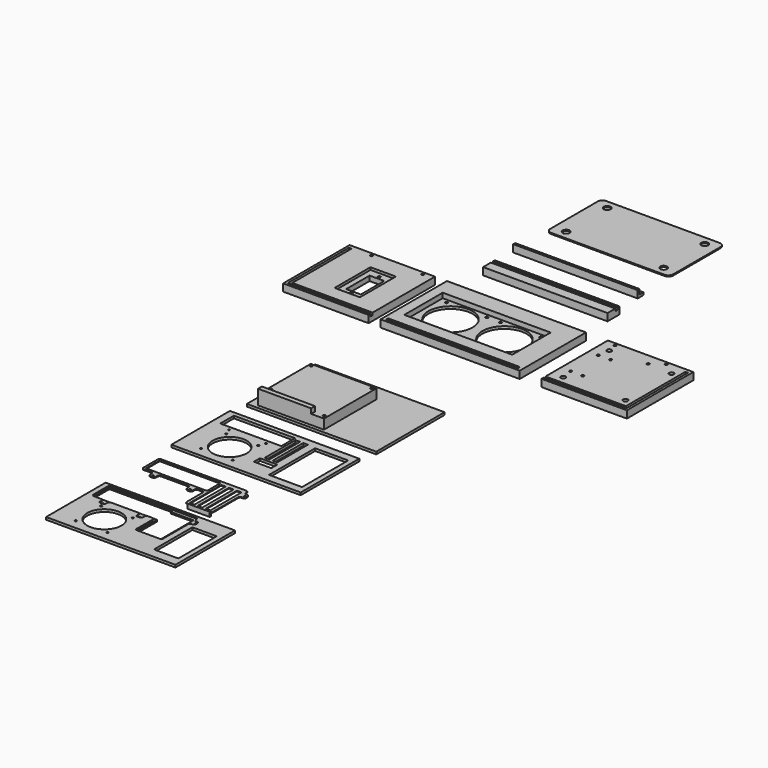
from build123d import *

# Parameters (mm, degrees)
F0_W      = 361.95
F0_H      = 215.9
F0_W_2    = 342.9
F0_H_2    = 6.731
F0_W_3    = 280.8
F0_H_3    = 125
F0_R      = 3.302
F0_R_2    = 57.5
F1_DEPTH  = 12.7
F2_DEPTH  = 6.35
F3_R      = 6
F3_R_2    = 3.302
F3_W      = 6.731
F3_H      = 3.556
F3_H_2    = 193.294
F4_DEPTH  = 12.7
F5_DEPTH  = 6.35
F6_R      = 3.302
F6_W      = 66.04
F6_H      = 116.84
F6_W_2    = 38.1
F6_H_2    = 76.2
F6_W_3    = 6.731
F6_H_3    = 193.294
F6_H_4    = 3.556
F7_DEPTH  = 12.7
F8_DEPTH  = 6.35
F9_DEPTH  = 6.35
F10_R     = 3.302
F10_W     = 138.0889187211
F10_H     = 12.6182494217
F11_DEPTH = 25.4
F12_DEPTH = 38.1
F13_R     = 3.302
F14_DEPTH = 6.4
F15_W     = 336.55
F15_H     = 190.385
F15_R     = 2.5
F15_R_2   = 44.5
F15_W_2   = 45.2000028
F15_H_2   = 20
F15_R_3   = 2.0970704069
F15_R_4   = 2.1817303996
F15_W_3   = 158.75
F15_H_3   = 44.45
F15_W_4   = 12.0000014
F15_H_4   = 99.38
F15_W_5   = 86
F15_H_5   = 150
F16_DEPTH = 6.3754
F17_W     = 323.85
F17_H     = 25.2222
F17_H_2   = 6.5278
F17_H_3   = 6.35
F18_DEPTH = 12.7
F19_DEPTH = 6.35
F20_R     = 9
F21_DEPTH = 3
F22_DEPTH = 6.35
F23_R     = 2
F23_W     = 158.75
F23_H     = 44.45
F24_DEPTH = 2
F25_DEPTH = 10
F26_W     = 336.55
F26_H     = 193.6500064
F26_R     = 2.5
F26_R_2   = 44.5
F26_W_2   = 63.5
F26_H_2   = 125
F26_R_3   = 2
F27_DEPTH = 6.4
F28_START = 4
F28_DEPTH = 2.4
F29_W     = 323.85
F29_H     = 6.35
F30_DEPTH = 19.05
F29_H_2   = 12.7
F31_DEPTH = 6.35


# Not quite as in the source:
# - a feature names something its author has since deleted; it is built from what else it names


with BuildPart() as f1:
    # F0 (on Top) → F1 (new body)
    with BuildSketch(Plane.XY):
        with Locations((-60.325, 0)):
            Rectangle(F0_W, F0_H)
        with Locations((-60.325, -98.2345)):
            Rectangle(F0_W_2, F0_H_2, mode=Mode.SUBTRACT)
        with Locations((-75.5, 0)):
            Rectangle(F0_W_3, F0_H_3, mode=Mode.SUBTRACT)
        with Locations((-60.325, -98.2345)):
            Rectangle(F0_W_2, F0_H_2)
        with Locations((-75.5, 0)):
            Rectangle(F0_W_3, F0_H_3)
        with Locations((-198.2, -52.5)):
            Circle(F0_R, mode=Mode.SUBTRACT)
        with Locations((-93.2, -52.5)):
            Circle(F0_R, mode=Mode.SUBTRACT)
        with Locations((-57.8, -52.5)):
            Circle(F0_R, mode=Mode.SUBTRACT)
        with Locations((47.2, -52.5)):
            Circle(F0_R, mode=Mode.SUBTRACT)
        with Locations((-198.2, 52.5)):
            Circle(F0_R, mode=Mode.SUBTRACT)
        with Locations((-145.7, 0)):
            Circle(F0_R_2, mode=Mode.SUBTRACT)
        with Locations((-93.2, 52.5)):
            Circle(F0_R, mode=Mode.SUBTRACT)
        with Locations((-5.3, 0)):
            Circle(F0_R_2, mode=Mode.SUBTRACT)
        with Locations((-57.8, 52.5)):
            Circle(F0_R, mode=Mode.SUBTRACT)
        with Locations((47.2, 52.5)):
            Circle(F0_R, mode=Mode.SUBTRACT)
    extrude(amount=-F1_DEPTH)

    # F0 (on Top) → F2 (join)
    with BuildSketch(Plane.XY):
        with Locations((-60.325, 0)):
            Rectangle(F0_W, F0_H)
        with Locations((-60.325, -98.2345)):
            Rectangle(F0_W_2, F0_H_2, mode=Mode.SUBTRACT)
        with Locations((-75.5, 0)):
            Rectangle(F0_W_3, F0_H_3, mode=Mode.SUBTRACT)
        with Locations((-75.5, 0)):
            Rectangle(F0_W_3, F0_H_3)
        with Locations((-198.2, -52.5)):
            Circle(F0_R, mode=Mode.SUBTRACT)
        with Locations((-93.2, -52.5)):
            Circle(F0_R, mode=Mode.SUBTRACT)
        with Locations((-57.8, -52.5)):
            Circle(F0_R, mode=Mode.SUBTRACT)
        with Locations((47.2, -52.5)):
            Circle(F0_R, mode=Mode.SUBTRACT)
        with Locations((-198.2, 52.5)):
            Circle(F0_R, mode=Mode.SUBTRACT)
        with Locations((-145.7, 0)):
            Circle(F0_R_2, mode=Mode.SUBTRACT)
        with Locations((-93.2, 52.5)):
            Circle(F0_R, mode=Mode.SUBTRACT)
        with Locations((-5.3, 0)):
            Circle(F0_R_2, mode=Mode.SUBTRACT)
        with Locations((-57.8, 52.5)):
            Circle(F0_R, mode=Mode.SUBTRACT)
        with Locations((47.2, 52.5)):
            Circle(F0_R, mode=Mode.SUBTRACT)
    extrude(amount=F2_DEPTH)

    # F0 (on Top) → F22 (cut, symmetric)
    with BuildSketch(Plane.XY):
        with Locations((-75.5, 0)):
            Rectangle(F0_W_3, F0_H_3)
        with Locations((-198.2, -52.5)):
            Circle(F0_R, mode=Mode.SUBTRACT)
        with Locations((-93.2, -52.5)):
            Circle(F0_R, mode=Mode.SUBTRACT)
        with Locations((-57.8, -52.5)):
            Circle(F0_R, mode=Mode.SUBTRACT)
        with Locations((47.2, -52.5)):
            Circle(F0_R, mode=Mode.SUBTRACT)
        with Locations((-198.2, 52.5)):
            Circle(F0_R, mode=Mode.SUBTRACT)
        with Locations((-145.7, 0)):
            Circle(F0_R_2, mode=Mode.SUBTRACT)
        with Locations((-93.2, 52.5)):
            Circle(F0_R, mode=Mode.SUBTRACT)
        with Locations((-5.3, 0)):
            Circle(F0_R_2, mode=Mode.SUBTRACT)
        with Locations((-57.8, 52.5)):
            Circle(F0_R, mode=Mode.SUBTRACT)
        with Locations((47.2, 52.5)):
            Circle(F0_R, mode=Mode.SUBTRACT)
    extrude(amount=F22_DEPTH, both=True, mode=Mode.SUBTRACT)


with BuildPart() as f4:
    # F3 (on Top) → F4 (new body)
    with BuildSketch(Plane.XY):
        Polygon((177.3511743546, -101.6), (177.3511743546, -107.95), (399.6011743546, -107.95), (399.6011743546, 107.95), (177.3511743546, 107.95), (177.3511743546, -94.869), (386.5201743546, -94.869), (386.5201743546, 98.425), (393.2511743546, 98.425), (393.2511743546, -94.869), (393.2511743546, -98.425), (393.2511743546, -101.6), align=None)
        with Locations((207.3511743546, -74.95)):
            Circle(F3_R, mode=Mode.SUBTRACT)
        with BuildLine():
            Line((231.2492377546, -45.0850025), (206.0531743546, -45.0850025))
            ThreePointArc((206.0531743546, -45.0850025), (200.4163077631, -47.4198690915), (202.7511743546, -41.7830025))
            Line((202.7511743546, -41.7830025), (202.7511743546, 41.7829975))
            ThreePointArc((202.7511743546, 41.7829975), (200.4163077631, 47.4198640915), (206.0531743546, 45.0849975))
            Line((206.0531743546, 45.0849975), (231.2492377546, 45.0849975))
            ThreePointArc((231.2492377546, 45.0849975), (234.5512377546, 48.3869975), (237.8532377546, 45.0849975))
            ThreePointArc((237.8532377546, 45.0849975), (236.886104346, 42.7501309085), (234.5512377546, 41.7829975))
            Line((234.5512377546, 41.7829975), (234.5512377546, -41.7830025))
            ThreePointArc((234.5512377546, -41.7830025), (236.886104346, -42.7501359085), (237.8532377546, -45.0850025))
            ThreePointArc((237.8532377546, -45.0850025), (234.5512377546, -48.3870025), (231.2492377546, -45.0850025))
        make_face(mode=Mode.SUBTRACT)
        with Locations((369.6011743546, -74.95)):
            Circle(F3_R, mode=Mode.SUBTRACT)
        with Locations((207.3511743546, 74.95)):
            Circle(F3_R, mode=Mode.SUBTRACT)
        with Locations((202.7511743546, 99.95)):
            Circle(F3_R_2, mode=Mode.SUBTRACT)
        with Locations((306.0201743546, 78.45)):
            Circle(F3_R_2, mode=Mode.SUBTRACT)
        with Locations((335.8979743546, 99.95)):
            Circle(F3_R_2, mode=Mode.SUBTRACT)
        with Locations((369.6011743546, 74.95)):
            Circle(F3_R, mode=Mode.SUBTRACT)
        Polygon((177.3511743546, -94.869), (177.3511743546, -101.6), (393.2511743546, -101.6), (393.2511743546, -98.425), (386.5201743546, -98.425), (386.5201743546, -94.869), align=None)
        with Locations((389.8856743546, -96.647)):
            Rectangle(F3_W, F3_H)
        with Locations((389.8856743546, 1.778)):
            Rectangle(F3_W, F3_H_2)
        with Locations((207.3511743546, 74.95)):
            Circle(F3_R)
        with Locations((207.3511743546, 74.95)):
            Circle(F3_R_2, mode=Mode.SUBTRACT)
        with Locations((207.3511743546, -74.95)):
            Circle(F3_R)
        with Locations((207.3511743546, -74.95)):
            Circle(F3_R_2, mode=Mode.SUBTRACT)
        with Locations((369.6011743546, -74.95)):
            Circle(F3_R)
        with Locations((369.6011743546, -74.95)):
            Circle(F3_R_2, mode=Mode.SUBTRACT)
        with Locations((369.6011743546, 74.95)):
            Circle(F3_R)
        with Locations((369.6011743546, 74.95)):
            Circle(F3_R_2, mode=Mode.SUBTRACT)
        with BuildLine():
            ThreePointArc((202.7511743546, -41.7830025), (205.086040946, -42.7501359085), (206.0531743546, -45.0850025))
            Line((206.0531743546, -45.0850025), (231.2492377546, -45.0850025))
            ThreePointArc((231.2492377546, -45.0850025), (232.2163711631, -42.7501359085), (234.5512377546, -41.7830025))
            Line((234.5512377546, -41.7830025), (234.5512377546, 41.7829975))
            ThreePointArc((234.5512377546, 41.7829975), (232.2163711631, 42.7501309085), (231.2492377546, 45.0849975))
            Line((231.2492377546, 45.0849975), (206.0531743546, 45.0849975))
            ThreePointArc((206.0531743546, 45.0849975), (205.086040946, 42.7501309085), (202.7511743546, 41.7829975))
            Line((202.7511743546, 41.7829975), (202.7511743546, -41.7830025))
        make_face()
    extrude(amount=-F4_DEPTH)

    # F3 (on Top) → F5 (join)
    with BuildSketch(Plane.XY):
        Polygon((177.3511743546, -101.6), (177.3511743546, -107.95), (399.6011743546, -107.95), (399.6011743546, 107.95), (177.3511743546, 107.95), (177.3511743546, -94.869), (386.5201743546, -94.869), (386.5201743546, 98.425), (393.2511743546, 98.425), (393.2511743546, -94.869), (393.2511743546, -98.425), (393.2511743546, -101.6), align=None)
        with Locations((207.3511743546, -74.95)):
            Circle(F3_R, mode=Mode.SUBTRACT)
        with BuildLine():
            Line((231.2492377546, -45.0850025), (206.0531743546, -45.0850025))
            ThreePointArc((206.0531743546, -45.0850025), (200.4163077631, -47.4198690915), (202.7511743546, -41.7830025))
            Line((202.7511743546, -41.7830025), (202.7511743546, 41.7829975))
            ThreePointArc((202.7511743546, 41.7829975), (200.4163077631, 47.4198640915), (206.0531743546, 45.0849975))
            Line((206.0531743546, 45.0849975), (231.2492377546, 45.0849975))
            ThreePointArc((231.2492377546, 45.0849975), (234.5512377546, 48.3869975), (237.8532377546, 45.0849975))
            ThreePointArc((237.8532377546, 45.0849975), (236.886104346, 42.7501309085), (234.5512377546, 41.7829975))
            Line((234.5512377546, 41.7829975), (234.5512377546, -41.7830025))
            ThreePointArc((234.5512377546, -41.7830025), (236.886104346, -42.7501359085), (237.8532377546, -45.0850025))
            ThreePointArc((237.8532377546, -45.0850025), (234.5512377546, -48.3870025), (231.2492377546, -45.0850025))
        make_face(mode=Mode.SUBTRACT)
        with Locations((369.6011743546, -74.95)):
            Circle(F3_R, mode=Mode.SUBTRACT)
        with Locations((207.3511743546, 74.95)):
            Circle(F3_R, mode=Mode.SUBTRACT)
        with Locations((202.7511743546, 99.95)):
            Circle(F3_R_2, mode=Mode.SUBTRACT)
        with Locations((306.0201743546, 78.45)):
            Circle(F3_R_2, mode=Mode.SUBTRACT)
        with Locations((335.8979743546, 99.95)):
            Circle(F3_R_2, mode=Mode.SUBTRACT)
        with Locations((369.6011743546, 74.95)):
            Circle(F3_R, mode=Mode.SUBTRACT)
        with BuildLine():
            ThreePointArc((202.7511743546, -41.7830025), (205.086040946, -42.7501359085), (206.0531743546, -45.0850025))
            Line((206.0531743546, -45.0850025), (231.2492377546, -45.0850025))
            ThreePointArc((231.2492377546, -45.0850025), (232.2163711631, -42.7501359085), (234.5512377546, -41.7830025))
            Line((234.5512377546, -41.7830025), (234.5512377546, 41.7829975))
            ThreePointArc((234.5512377546, 41.7829975), (232.2163711631, 42.7501309085), (231.2492377546, 45.0849975))
            Line((231.2492377546, 45.0849975), (206.0531743546, 45.0849975))
            ThreePointArc((206.0531743546, 45.0849975), (205.086040946, 42.7501309085), (202.7511743546, 41.7829975))
            Line((202.7511743546, 41.7829975), (202.7511743546, -41.7830025))
        make_face()
    extrude(amount=F5_DEPTH)


with BuildPart() as f7:
    # F6 (on Top) → F7 (new body)
    with BuildSketch(Plane.XY):
        Polygon((-272.3593753815, -94.869), (-272.3593753815, 107.95), (-494.6093753815, 107.95), (-494.6093753815, -107.95), (-272.3593753815, -107.95), (-272.3593753815, -101.6), (-488.2593753815, -101.6), (-488.2593753815, -98.425), (-488.2593753815, -94.869), (-488.2593753815, 98.425), (-481.5283753815, 98.425), (-481.5283753815, -94.869), align=None)
        with Locations((-430.9061753815, 99.95)):
            Circle(F6_R, mode=Mode.SUBTRACT)
        with Locations((-367.6093753815, 0)):
            Rectangle(F6_W, F6_H, mode=Mode.SUBTRACT)
        with Locations((-297.7593753815, 99.95)):
            Circle(F6_R, mode=Mode.SUBTRACT)
        with Locations((-367.6093753815, 0)):
            Rectangle(F6_W, F6_H)
        with Locations((-367.6093753815, -45.6)):
            Circle(F6_R, mode=Mode.SUBTRACT)
        with Locations((-367.6093753815, 0)):
            Rectangle(F6_W_2, F6_H_2, mode=Mode.SUBTRACT)
        with Locations((-367.6093753815, 45.6)):
            Circle(F6_R, mode=Mode.SUBTRACT)
        Polygon((-272.3593753815, -101.6), (-272.3593753815, -94.869), (-481.5283753815, -94.869), (-481.5283753815, -98.425), (-488.2593753815, -98.425), (-488.2593753815, -101.6), align=None)
        with Locations((-484.8938753815, 1.778)):
            Rectangle(F6_W_3, F6_H_3)
        with Locations((-484.8938753815, -96.647)):
            Rectangle(F6_W_3, F6_H_4)
    extrude(amount=-F7_DEPTH)

    # F6 (on Top) → F8 (join)
    with BuildSketch(Plane.XY):
        Polygon((-272.3593753815, -94.869), (-272.3593753815, 107.95), (-494.6093753815, 107.95), (-494.6093753815, -107.95), (-272.3593753815, -107.95), (-272.3593753815, -101.6), (-488.2593753815, -101.6), (-488.2593753815, -98.425), (-488.2593753815, -94.869), (-488.2593753815, 98.425), (-481.5283753815, 98.425), (-481.5283753815, -94.869), align=None)
        with Locations((-430.9061753815, 99.95)):
            Circle(F6_R, mode=Mode.SUBTRACT)
        with Locations((-367.6093753815, 0)):
            Rectangle(F6_W, F6_H, mode=Mode.SUBTRACT)
        with Locations((-297.7593753815, 99.95)):
            Circle(F6_R, mode=Mode.SUBTRACT)
        with Locations((-367.6093753815, 0)):
            Rectangle(F6_W, F6_H)
        with Locations((-367.6093753815, -45.6)):
            Circle(F6_R, mode=Mode.SUBTRACT)
        with Locations((-367.6093753815, 0)):
            Rectangle(F6_W_2, F6_H_2, mode=Mode.SUBTRACT)
        with Locations((-367.6093753815, 45.6)):
            Circle(F6_R, mode=Mode.SUBTRACT)
    extrude(amount=F8_DEPTH)

    # F6 (on Top) → F9 (cut)
    with BuildSketch(Plane.XY):
        with Locations((-367.6093753815, 0)):
            Rectangle(F6_W, F6_H)
        with Locations((-367.6093753815, -45.6)):
            Circle(F6_R, mode=Mode.SUBTRACT)
        with Locations((-367.6093753815, 0)):
            Rectangle(F6_W_2, F6_H_2, mode=Mode.SUBTRACT)
        with Locations((-367.6093753815, 45.6)):
            Circle(F6_R, mode=Mode.SUBTRACT)
    extrude(amount=F9_DEPTH, mode=Mode.SUBTRACT)


with BuildPart() as f11:
    # F10 (on Top) → F11 (new body)
    with BuildSketch(Plane.XY):
        Polygon((-35.35, -549.4468963333), (-35.35, -377.9968963333), (-206.8, -377.9968963333), (-206.8, -536.8286469116), (-68.7110812789, -536.8286469116), (-68.7110812789, -549.4468963333), align=None)
        with Locations((-200.45, -516.4268963333)):
            Circle(F10_R, mode=Mode.SUBTRACT)
        with Locations((-42.97, -539.2868963333)):
            Circle(F10_R, mode=Mode.SUBTRACT)
        with Locations((-200.45, -384.3468963333)):
            Circle(F10_R, mode=Mode.SUBTRACT)
        with Locations((-42.97, -384.3468963333)):
            Circle(F10_R, mode=Mode.SUBTRACT)
        with Locations((-137.7555406395, -543.1377716225)):
            Rectangle(F10_W, F10_H)
    extrude(amount=F11_DEPTH)

    # F10 (on Top) → F12 (join)
    with BuildSketch(Plane.XY):
        with Locations((-137.7555406395, -543.1377716225)):
            Rectangle(F10_W, F10_H)
    extrude(amount=F12_DEPTH)


with BuildPart() as f14:
    # F13 (on Top) → F14 (new body)
    with BuildSketch(Plane.XY):
        Polygon((107.95, -558.4746963333), (107.95, -336.2246963333), (-228.6, -336.2246963333), (-228.6, -551.9468963333), (-228.6, -558.4746963333), align=None)
        with Locations((-200.45, -516.4268963333)):
            Circle(F13_R, mode=Mode.SUBTRACT)
        with Locations((-42.97, -539.2868963333)):
            Circle(F13_R, mode=Mode.SUBTRACT)
        with Locations((-200.45, -384.3468963333)):
            Circle(F13_R, mode=Mode.SUBTRACT)
        with Locations((-42.97, -384.3468963333)):
            Circle(F13_R, mode=Mode.SUBTRACT)
    extrude(amount=-F14_DEPTH)


with BuildPart() as f16:
    # F15 (on Top) → F16 (new body)
    with BuildSketch(Plane.XY):
        with Locations((-60.325, -708.9570045471)):
            Rectangle(F15_W, F15_H)
        with Locations((-171.0694, -779.3595045471)):
            Circle(F15_R, mode=Mode.SUBTRACT)
        with Locations((-88.5694, -779.3595045471)):
            Circle(F15_R, mode=Mode.SUBTRACT)
        with Locations((-129.8194, -738.1095045471)):
            Circle(F15_R_2, mode=Mode.SUBTRACT)
        with Locations((-28.20002274, -747.9644930071)):
            Rectangle(F15_W_2, F15_H_2, mode=Mode.SUBTRACT)
        with Locations((-171.0694, -696.8595045471)):
            Circle(F15_R, mode=Mode.SUBTRACT)
        with Locations((-177.92501754, -679.9145094071)):
            Circle(F15_R_3, mode=Mode.SUBTRACT)
        with Locations((-88.5694, -696.8595045471)):
            Circle(F15_R, mode=Mode.SUBTRACT)
        with Locations((-81.72500674, -679.9145094071)):
            Circle(F15_R_4, mode=Mode.SUBTRACT)
        with Locations((-129.82501214, -647.1895050071)):
            Rectangle(F15_W_3, F15_H_3, mode=Mode.SUBTRACT)
        with Locations((-38.45002344, -680.6544930071)):
            Rectangle(F15_W_4, F15_H_4, mode=Mode.SUBTRACT)
        with Locations((-17.95002204, -680.6544930071)):
            Rectangle(F15_W_4, F15_H_4, mode=Mode.SUBTRACT)
        with Locations((52.25, -708.9570045471)):
            Rectangle(F15_W_5, F15_H_5, mode=Mode.SUBTRACT)
    extrude(amount=F16_DEPTH)


with BuildPart() as f18:
    # F17 (on Top) → F18 (new body)
    with BuildSketch(Plane.XY):
        with Locations((-60.325, 214.3075841795)):
            Rectangle(F17_W, F17_H)
        with Locations((-60.325, 230.1825841795)):
            Rectangle(F17_W, F17_H_2)
        with Locations((-60.325, 236.6214841795)):
            Rectangle(F17_W, F17_H_3)
    extrude(amount=-F18_DEPTH)

    # F17 (on Top) → F19 (join)
    with BuildSketch(Plane.XY):
        with Locations((-60.325, 236.6214841795)):
            Rectangle(F17_W, F17_H_3)
        with Locations((-60.325, 214.3075841795)):
            Rectangle(F17_W, F17_H)
    extrude(amount=F19_DEPTH)


with BuildPart() as f21:
    # F20 (on Top) → F21 (new body)
    with BuildSketch(Plane.XY):
        with BuildLine():
            ThreePointArc((-224.79, 423.5097664064), (-221.0702561211, 414.5295102853), (-212.09, 410.8097664064))
            Line((-212.09, 410.8097664064), (82.4, 410.8097664064))
            ThreePointArc((82.4, 410.8097664064), (91.3802561211, 414.5295102853), (95.1, 423.5097664064))
            Line((95.1, 423.5097664064), (95.1, 577.3067664064))
            ThreePointArc((95.1, 577.3067664064), (91.3802561211, 586.2870225275), (82.4, 590.0067664064))
            Line((82.4, 590.0067664064), (-212.09, 590.0067664064))
            ThreePointArc((-212.09, 590.0067664064), (-221.0702561211, 586.2870225275), (-224.79, 577.3067664064))
            Line((-224.79, 577.3067664064), (-224.79, 423.5097664064))
        make_face()
        with Locations((-191.77, 433.6697664064)):
            Circle(F20_R, mode=Mode.SUBTRACT)
        with Locations((62.08, 433.6697664064)):
            Circle(F20_R, mode=Mode.SUBTRACT)
        with Locations((-191.77, 567.1467664064)):
            Circle(F20_R, mode=Mode.SUBTRACT)
        with Locations((62.08, 567.1467664064)):
            Circle(F20_R, mode=Mode.SUBTRACT)
    extrude(amount=F21_DEPTH)


with BuildPart() as f24:
    # F23 (on Top) → F24 (new body)
    with BuildSketch(Plane.XY):
        with BuildLine():
            Line((-3.45002134, -872.449751843), (8.54998006, -872.449751843))
            Line((8.54998006, -872.449751843), (8.54998006, -974.0499811521))
            Line((8.54998006, -974.0499811521), (11.08998006, -974.0499811521))
            Line((11.08998006, -974.0499811521), (11.08998006, -979.449751843))
            Line((11.08998006, -979.449751843), (11.46998006, -979.449751843))
            ThreePointArc((11.46998006, -979.449751843), (15.0620825084, -977.9618542914), (16.54998006, -974.369751843))
            Line((16.54998006, -974.369751843), (16.54998006, -893.4699931521))
            ThreePointArc((16.54998006, -893.4699931521), (18.0378776116, -889.8778907037), (21.62998006, -888.3899931521))
            Line((21.62998006, -888.3899931521), (24.16998006, -888.3899931521))
            ThreePointArc((24.16998006, -888.3899931521), (27.7620825084, -886.9020956005), (29.24998006, -883.3099931521))
            Line((29.24998006, -883.3099931521), (29.24998006, -878.2299931521))
            ThreePointArc((29.24998006, -878.2299931521), (27.7620825084, -874.6378907037), (24.16998006, -873.1499931521))
            Line((24.16998006, -873.1499931521), (21.62998006, -873.1499931521))
            ThreePointArc((21.62998006, -873.1499931521), (18.0378776116, -871.6620956005), (16.54998006, -868.0699931521))
            Line((16.54998006, -868.0699931521), (16.54998006, -865.5299931521))
            ThreePointArc((16.54998006, -865.5299931521), (15.0620825084, -861.9378907037), (11.46998006, -860.4499931521))
            Line((11.46998006, -860.4499931521), (-210.12001214, -860.4499931521))
            ThreePointArc((-210.12001214, -860.4499931521), (-213.7121145884, -861.9378907037), (-215.20001214, -865.5299931521))
            Line((-215.20001214, -865.5299931521), (-215.20001214, -911.8199931521))
            ThreePointArc((-215.20001214, -911.8199931521), (-213.7121145884, -915.4120956005), (-210.12001214, -916.8999931521))
            Line((-210.12001214, -916.8999931521), (-190.62501754, -916.8999931521))
            ThreePointArc((-190.62501754, -916.8999931521), (-187.0329150916, -918.3878907037), (-185.54501754, -921.9799931521))
            Line((-185.54501754, -921.9799931521), (-185.54501754, -927.0599931521))
            ThreePointArc((-185.54501754, -927.0599931521), (-184.0571199884, -930.6520956005), (-180.46501754, -932.1399931521))
            Line((-180.46501754, -932.1399931521), (-175.38501754, -932.1399931521))
            ThreePointArc((-175.38501754, -932.1399931521), (-171.7929150916, -930.6520956005), (-170.30501754, -927.0599931521))
            Line((-170.30501754, -927.0599931521), (-170.30501754, -921.9799931521))
            ThreePointArc((-170.30501754, -921.9799931521), (-168.8171199884, -918.3878907037), (-165.22501754, -916.8999931521))
            Line((-165.22501754, -916.8999931521), (-94.42500674, -916.8999931521))
            ThreePointArc((-94.42500674, -916.8999931521), (-90.8329042916, -918.3878907037), (-89.34500674, -921.9799931521))
            Line((-89.34500674, -921.9799931521), (-89.34500674, -927.0599931521))
            ThreePointArc((-89.34500674, -927.0599931521), (-87.8571091884, -930.6520956005), (-84.26500674, -932.1399931521))
            Line((-84.26500674, -932.1399931521), (-79.18500674, -932.1399931521))
            ThreePointArc((-79.18500674, -932.1399931521), (-75.5929042916, -930.6520956005), (-74.10500674, -927.0599931521))
            Line((-74.10500674, -927.0599931521), (-74.10500674, -921.9799931521))
            ThreePointArc((-74.10500674, -921.9799931521), (-72.6171091884, -918.3878907037), (-69.02500674, -916.8999931521))
            Line((-69.02500674, -916.8999931521), (-57.53002414, -916.8999931521))
            ThreePointArc((-57.53002414, -916.8999931521), (-53.9379216916, -918.3878907037), (-52.45002414, -921.9799931521))
            Line((-52.45002414, -921.9799931521), (-52.45002414, -974.369751843))
            ThreePointArc((-52.45002414, -974.369751843), (-50.9621265884, -977.9618542914), (-47.37002414, -979.449751843))
            Line((-47.37002414, -979.449751843), (-46.99002414, -979.449751843))
            Line((-46.99002414, -979.449751843), (-46.99002414, -974.0499811521))
            Line((-46.99002414, -974.0499811521), (-44.45002414, -974.0499811521))
            Line((-44.45002414, -974.0499811521), (-44.45002414, -872.4499811521))
            Line((-44.45002414, -872.4499811521), (-32.45002274, -872.4499811521))
            Line((-32.45002274, -872.4499811521), (-32.45002274, -974.0499811521))
            Line((-32.45002274, -974.0499811521), (-23.95002274, -974.0499811521))
            Line((-23.95002274, -974.0499811521), (-23.95002274, -872.4499811521))
            Line((-23.95002274, -872.4499811521), (-11.95002134, -872.4499811521))
            Line((-11.95002134, -872.4499811521), (-11.95002134, -974.0499811521))
            Line((-11.95002134, -974.0499811521), (-3.45002134, -974.0499811521))
            Line((-3.45002134, -974.0499811521), (-3.45002134, -872.449751843))
        make_face()
        with Locations((-177.92501754, -927.4099931521)):
            Circle(F23_R, mode=Mode.SUBTRACT)
        with Locations((-81.72500674, -927.4099931521)):
            Circle(F23_R, mode=Mode.SUBTRACT)
        with Locations((-129.82501214, -888.6749931521)):
            Rectangle(F23_W, F23_H, mode=Mode.SUBTRACT)
        with Locations((24.51999206, -880.7699931521)):
            Circle(F23_R, mode=Mode.SUBTRACT)
        Polygon((11.08998006, -974.0499811521), (8.54998006, -974.0499811521), (-3.45002134, -974.0499811521), (-11.95002134, -974.0499811521), (-23.95002274, -974.0499811521), (-32.45002274, -974.0499811521), (-44.45002414, -974.0499811521), (-46.99002414, -974.0499811521), (-46.99002414, -979.449751843), (11.08998006, -979.449751843), align=None)
    extrude(amount=F24_DEPTH)

    # F23 (on Top) → F25 (join)
    with BuildSketch(Plane.XY):
        Polygon((11.08998006, -974.0499811521), (8.54998006, -974.0499811521), (-3.45002134, -974.0499811521), (-11.95002134, -974.0499811521), (-23.95002274, -974.0499811521), (-32.45002274, -974.0499811521), (-44.45002414, -974.0499811521), (-46.99002414, -974.0499811521), (-46.99002414, -979.449751843), (11.08998006, -979.449751843), align=None)
    extrude(amount=-F25_DEPTH)


with BuildPart() as f27:
    # F26 (on Top) → F27 (new body)
    with BuildSketch(Plane.XY):
        with Locations((-60.325, -1114.7701744505)):
            Rectangle(F26_W, F26_H)
        with Locations((-171.0694, -1186.8051776505)):
            Circle(F26_R, mode=Mode.SUBTRACT)
        with Locations((-88.5694, -1186.8054069595)):
            Circle(F26_R, mode=Mode.SUBTRACT)
        with Locations((-129.8194, -1145.5551776505)):
            Circle(F26_R_2, mode=Mode.SUBTRACT)
        with Locations((63.5, -1123.6951776505)):
            Rectangle(F26_W_2, F26_H_2, mode=Mode.SUBTRACT)
        with Locations((-171.0694, -1104.3049483414)):
            Circle(F26_R, mode=Mode.SUBTRACT)
        with Locations((-88.5694, -1104.3051776505)):
            Circle(F26_R, mode=Mode.SUBTRACT)
        with BuildLine():
            Line((11.46998006, -1142.1449304014), (11.08998006, -1142.1449304014))
            Line((11.08998006, -1142.1449304014), (-46.99002414, -1142.1449304014))
            Line((-46.99002414, -1142.1449304014), (-47.37002414, -1142.1449304014))
            ThreePointArc((-47.37002414, -1142.1449304014), (-50.9621265884, -1140.6570328498), (-52.45002414, -1137.0649304014))
            Line((-52.45002414, -1137.0649304014), (-52.45002414, -1084.6751717105))
            ThreePointArc((-52.45002414, -1084.6751717105), (-53.9379216916, -1081.083069262), (-57.53002414, -1079.5951717105))
            Line((-57.53002414, -1079.5951717105), (-69.02500674, -1079.5951717105))
            ThreePointArc((-69.02500674, -1079.5951717105), (-72.6171091884, -1081.083069262), (-74.10500674, -1084.6751717105))
            Line((-74.10500674, -1084.6751717105), (-74.10500674, -1089.7551717105))
            ThreePointArc((-74.10500674, -1089.7551717105), (-75.5929042916, -1093.3472741589), (-79.18500674, -1094.8351717105))
            Line((-79.18500674, -1094.8351717105), (-84.26500674, -1094.8351717105))
            ThreePointArc((-84.26500674, -1094.8351717105), (-87.8571091884, -1093.3472741589), (-89.34500674, -1089.7551717105))
            Line((-89.34500674, -1089.7551717105), (-89.34500674, -1084.6751717105))
            ThreePointArc((-89.34500674, -1084.6751717105), (-90.8329042916, -1081.083069262), (-94.42500674, -1079.5951717105))
            Line((-94.42500674, -1079.5951717105), (-165.22501754, -1079.5951717105))
            ThreePointArc((-165.22501754, -1079.5951717105), (-168.8171199884, -1081.083069262), (-170.30501754, -1084.6751717105))
            Line((-170.30501754, -1084.6751717105), (-170.30501754, -1089.7551717105))
            ThreePointArc((-170.30501754, -1089.7551717105), (-171.7929150916, -1093.3472741589), (-175.38501754, -1094.8351717105))
            Line((-175.38501754, -1094.8351717105), (-180.46501754, -1094.8351717105))
            ThreePointArc((-180.46501754, -1094.8351717105), (-184.0571199884, -1093.3472741589), (-185.54501754, -1089.7551717105))
            Line((-185.54501754, -1089.7551717105), (-185.54501754, -1084.656734079))
            ThreePointArc((-185.54501754, -1084.656734079), (-187.0329150916, -1081.0646316305), (-190.62501754, -1079.576734079))
            Line((-190.62501754, -1079.576734079), (-210.12001214, -1079.576734079))
            ThreePointArc((-210.12001214, -1079.576734079), (-213.7121145884, -1078.0888365274), (-215.20001214, -1074.496734079))
            Line((-215.20001214, -1074.496734079), (-215.20001214, -1028.2251717105))
            ThreePointArc((-215.20001214, -1028.2251717105), (-213.7121145884, -1024.633069262), (-210.12001214, -1023.1451717105))
            Line((-210.12001214, -1023.1451717105), (11.46998006, -1023.1451717105))
            ThreePointArc((11.46998006, -1023.1451717105), (15.0620825084, -1024.633069262), (16.54998006, -1028.2251717105))
            Line((16.54998006, -1028.2251717105), (16.54998006, -1030.7651717105))
            ThreePointArc((16.54998006, -1030.7651717105), (18.0378776116, -1034.3572741589), (21.62998006, -1035.8451717105))
            Line((21.62998006, -1035.8451717105), (24.16998006, -1035.8451717105))
            ThreePointArc((24.16998006, -1035.8451717105), (27.7620825084, -1037.333069262), (29.24998006, -1040.9251717105))
            Line((29.24998006, -1040.9251717105), (29.24998006, -1046.0051717105))
            ThreePointArc((29.24998006, -1046.0051717105), (27.7620825084, -1049.5972741589), (24.16998006, -1051.0851717105))
            Line((24.16998006, -1051.0851717105), (21.62998006, -1051.0851717105))
            ThreePointArc((21.62998006, -1051.0851717105), (18.0378776116, -1052.573069262), (16.54998006, -1056.1651717105))
            Line((16.54998006, -1056.1651717105), (16.54998006, -1137.0649304014))
            ThreePointArc((16.54998006, -1137.0649304014), (15.0620825084, -1140.6570328498), (11.46998006, -1142.1449304014))
        make_face(mode=Mode.SUBTRACT)
        with BuildLine():
            Line((11.54998006, -1136.7451597105), (11.08998006, -1136.7451597105))
            Line((11.08998006, -1136.7451597105), (11.08998006, -1142.1449304014))
            Line((11.08998006, -1142.1449304014), (11.46998006, -1142.1449304014))
            ThreePointArc((11.46998006, -1142.1449304014), (15.0620825084, -1140.6570328498), (16.54998006, -1137.0649304014))
            Line((16.54998006, -1137.0649304014), (16.54998006, -1056.1651717105))
            ThreePointArc((16.54998006, -1056.1651717105), (18.0378776116, -1052.573069262), (21.62998006, -1051.0851717105))
            Line((21.62998006, -1051.0851717105), (24.16998006, -1051.0851717105))
            ThreePointArc((24.16998006, -1051.0851717105), (27.7620825084, -1049.5972741589), (29.24998006, -1046.0051717105))
            Line((29.24998006, -1046.0051717105), (29.24998006, -1040.9251717105))
            ThreePointArc((29.24998006, -1040.9251717105), (27.7620825084, -1037.333069262), (24.16998006, -1035.8451717105))
            Line((24.16998006, -1035.8451717105), (21.62998006, -1035.8451717105))
            ThreePointArc((21.62998006, -1035.8451717105), (18.0378776116, -1034.3572741589), (16.54998006, -1030.7651717105))
            Line((16.54998006, -1030.7651717105), (16.54998006, -1028.2251717105))
            ThreePointArc((16.54998006, -1028.2251717105), (15.0620825084, -1024.633069262), (11.46998006, -1023.1451717105))
            Line((11.46998006, -1023.1451717105), (-210.12001214, -1023.1451717105))
            ThreePointArc((-210.12001214, -1023.1451717105), (-213.7121145884, -1024.633069262), (-215.20001214, -1028.2251717105))
            Line((-215.20001214, -1028.2251717105), (-215.20001214, -1074.496734079))
            ThreePointArc((-215.20001214, -1074.496734079), (-213.7121145884, -1078.0888365274), (-210.12001214, -1079.576734079))
            Line((-210.12001214, -1079.576734079), (-190.62501754, -1079.576734079))
            ThreePointArc((-190.62501754, -1079.576734079), (-187.0329150916, -1081.0646316305), (-185.54501754, -1084.656734079))
            Line((-185.54501754, -1084.656734079), (-185.54501754, -1089.7551717105))
            ThreePointArc((-185.54501754, -1089.7551717105), (-184.0571199884, -1093.3472741589), (-180.46501754, -1094.8351717105))
            Line((-180.46501754, -1094.8351717105), (-175.38501754, -1094.8351717105))
            ThreePointArc((-175.38501754, -1094.8351717105), (-171.7929150916, -1093.3472741589), (-170.30501754, -1089.7551717105))
            Line((-170.30501754, -1089.7551717105), (-170.30501754, -1084.6751717105))
            ThreePointArc((-170.30501754, -1084.6751717105), (-168.8171199884, -1081.083069262), (-165.22501754, -1079.5951717105))
            Line((-165.22501754, -1079.5951717105), (-94.42500674, -1079.5951717105))
            ThreePointArc((-94.42500674, -1079.5951717105), (-90.8329042916, -1081.083069262), (-89.34500674, -1084.6751717105))
            Line((-89.34500674, -1084.6751717105), (-89.34500674, -1089.7551717105))
            ThreePointArc((-89.34500674, -1089.7551717105), (-87.8571091884, -1093.3472741589), (-84.26500674, -1094.8351717105))
            Line((-84.26500674, -1094.8351717105), (-79.18500674, -1094.8351717105))
            ThreePointArc((-79.18500674, -1094.8351717105), (-75.5929042916, -1093.3472741589), (-74.10500674, -1089.7551717105))
            Line((-74.10500674, -1089.7551717105), (-74.10500674, -1084.6751717105))
            ThreePointArc((-74.10500674, -1084.6751717105), (-72.6171091884, -1081.083069262), (-69.02500674, -1079.5951717105))
            Line((-69.02500674, -1079.5951717105), (-57.53002414, -1079.5951717105))
            ThreePointArc((-57.53002414, -1079.5951717105), (-53.9379216916, -1081.083069262), (-52.45002414, -1084.6751717105))
            Line((-52.45002414, -1084.6751717105), (-52.45002414, -1137.0649304014))
            ThreePointArc((-52.45002414, -1137.0649304014), (-50.9621265884, -1140.6570328498), (-47.37002414, -1142.1449304014))
            Line((-47.37002414, -1142.1449304014), (-46.99002414, -1142.1449304014))
            Line((-46.99002414, -1142.1449304014), (-46.99002414, -1136.7451597105))
            Line((-46.99002414, -1136.7451597105), (-47.45001214, -1136.7451597105))
            Line((-47.45001214, -1136.7451597105), (-47.45001214, -1076.5951717105))
            Line((-47.45001214, -1076.5951717105), (-212.20001214, -1076.5951717105))
            Line((-212.20001214, -1076.5951717105), (-212.20001214, -1026.1451717105))
            Line((-212.20001214, -1026.1451717105), (-47.45001214, -1026.1451717105))
            Line((-47.45001214, -1026.1451717105), (-47.45001214, -1032.1451597105))
            Line((-47.45001214, -1032.1451597105), (11.54998006, -1032.1451597105))
            Line((11.54998006, -1032.1451597105), (11.54998006, -1136.7451597105))
        make_face()
        with Locations((-177.92501754, -1090.1051717105)):
            Circle(F26_R_3, mode=Mode.SUBTRACT)
        with Locations((-81.72500674, -1090.1051717105)):
            Circle(F26_R_3, mode=Mode.SUBTRACT)
        with Locations((24.51999206, -1043.4651717105)):
            Circle(F26_R_3, mode=Mode.SUBTRACT)
    extrude(amount=F27_DEPTH)

    # F26 (on Top) → F28 (cut)
    with BuildSketch(Plane.XY.offset(F28_START)):
        with BuildLine():
            Line((11.54998006, -1136.7451597105), (11.08998006, -1136.7451597105))
            Line((11.08998006, -1136.7451597105), (11.08998006, -1142.1449304014))
            Line((11.08998006, -1142.1449304014), (11.46998006, -1142.1449304014))
            ThreePointArc((11.46998006, -1142.1449304014), (15.0620825084, -1140.6570328498), (16.54998006, -1137.0649304014))
            Line((16.54998006, -1137.0649304014), (16.54998006, -1056.1651717105))
            ThreePointArc((16.54998006, -1056.1651717105), (18.0378776116, -1052.573069262), (21.62998006, -1051.0851717105))
            Line((21.62998006, -1051.0851717105), (24.16998006, -1051.0851717105))
            ThreePointArc((24.16998006, -1051.0851717105), (27.7620825084, -1049.5972741589), (29.24998006, -1046.0051717105))
            Line((29.24998006, -1046.0051717105), (29.24998006, -1040.9251717105))
            ThreePointArc((29.24998006, -1040.9251717105), (27.7620825084, -1037.333069262), (24.16998006, -1035.8451717105))
            Line((24.16998006, -1035.8451717105), (21.62998006, -1035.8451717105))
            ThreePointArc((21.62998006, -1035.8451717105), (18.0378776116, -1034.3572741589), (16.54998006, -1030.7651717105))
            Line((16.54998006, -1030.7651717105), (16.54998006, -1028.2251717105))
            ThreePointArc((16.54998006, -1028.2251717105), (15.0620825084, -1024.633069262), (11.46998006, -1023.1451717105))
            Line((11.46998006, -1023.1451717105), (-210.12001214, -1023.1451717105))
            ThreePointArc((-210.12001214, -1023.1451717105), (-213.7121145884, -1024.633069262), (-215.20001214, -1028.2251717105))
            Line((-215.20001214, -1028.2251717105), (-215.20001214, -1074.496734079))
            ThreePointArc((-215.20001214, -1074.496734079), (-213.7121145884, -1078.0888365274), (-210.12001214, -1079.576734079))
            Line((-210.12001214, -1079.576734079), (-190.62501754, -1079.576734079))
            ThreePointArc((-190.62501754, -1079.576734079), (-187.0329150916, -1081.0646316305), (-185.54501754, -1084.656734079))
            Line((-185.54501754, -1084.656734079), (-185.54501754, -1089.7551717105))
            ThreePointArc((-185.54501754, -1089.7551717105), (-184.0571199884, -1093.3472741589), (-180.46501754, -1094.8351717105))
            Line((-180.46501754, -1094.8351717105), (-175.38501754, -1094.8351717105))
            ThreePointArc((-175.38501754, -1094.8351717105), (-171.7929150916, -1093.3472741589), (-170.30501754, -1089.7551717105))
            Line((-170.30501754, -1089.7551717105), (-170.30501754, -1084.6751717105))
            ThreePointArc((-170.30501754, -1084.6751717105), (-168.8171199884, -1081.083069262), (-165.22501754, -1079.5951717105))
            Line((-165.22501754, -1079.5951717105), (-94.42500674, -1079.5951717105))
            ThreePointArc((-94.42500674, -1079.5951717105), (-90.8329042916, -1081.083069262), (-89.34500674, -1084.6751717105))
            Line((-89.34500674, -1084.6751717105), (-89.34500674, -1089.7551717105))
            ThreePointArc((-89.34500674, -1089.7551717105), (-87.8571091884, -1093.3472741589), (-84.26500674, -1094.8351717105))
            Line((-84.26500674, -1094.8351717105), (-79.18500674, -1094.8351717105))
            ThreePointArc((-79.18500674, -1094.8351717105), (-75.5929042916, -1093.3472741589), (-74.10500674, -1089.7551717105))
            Line((-74.10500674, -1089.7551717105), (-74.10500674, -1084.6751717105))
            ThreePointArc((-74.10500674, -1084.6751717105), (-72.6171091884, -1081.083069262), (-69.02500674, -1079.5951717105))
            Line((-69.02500674, -1079.5951717105), (-57.53002414, -1079.5951717105))
            ThreePointArc((-57.53002414, -1079.5951717105), (-53.9379216916, -1081.083069262), (-52.45002414, -1084.6751717105))
            Line((-52.45002414, -1084.6751717105), (-52.45002414, -1137.0649304014))
            ThreePointArc((-52.45002414, -1137.0649304014), (-50.9621265884, -1140.6570328498), (-47.37002414, -1142.1449304014))
            Line((-47.37002414, -1142.1449304014), (-46.99002414, -1142.1449304014))
            Line((-46.99002414, -1142.1449304014), (-46.99002414, -1136.7451597105))
            Line((-46.99002414, -1136.7451597105), (-47.45001214, -1136.7451597105))
            Line((-47.45001214, -1136.7451597105), (-47.45001214, -1076.5951717105))
            Line((-47.45001214, -1076.5951717105), (-212.20001214, -1076.5951717105))
            Line((-212.20001214, -1076.5951717105), (-212.20001214, -1026.1451717105))
            Line((-212.20001214, -1026.1451717105), (-47.45001214, -1026.1451717105))
            Line((-47.45001214, -1026.1451717105), (-47.45001214, -1032.1451597105))
            Line((-47.45001214, -1032.1451597105), (11.54998006, -1032.1451597105))
            Line((11.54998006, -1032.1451597105), (11.54998006, -1136.7451597105))
        make_face()
        with Locations((-177.92501754, -1090.1051717105)):
            Circle(F26_R_3, mode=Mode.SUBTRACT)
        with Locations((-81.72500674, -1090.1051717105)):
            Circle(F26_R_3, mode=Mode.SUBTRACT)
        with Locations((24.51999206, -1043.4651717105)):
            Circle(F26_R_3, mode=Mode.SUBTRACT)
    extrude(amount=F28_DEPTH, mode=Mode.SUBTRACT)


with BuildPart() as f30:
    # F29 (on Top) → F30 (new body)
    with BuildSketch(Plane.XY):
        with Locations((-60.325, 302.708096838)):
            Rectangle(F29_W, F29_H)
    extrude(amount=F30_DEPTH)

    # F29 (on Top) → F31 (join)
    with BuildSketch(Plane.XY):
        with Locations((-60.325, 312.233096838)):
            Rectangle(F29_W, F29_H_2)
    extrude(amount=F31_DEPTH)


solid = Compound([f1.part, f4.part, f7.part, f11.part, f14.part, f16.part, f18.part, f21.part, f24.part, f27.part, f30.part])
